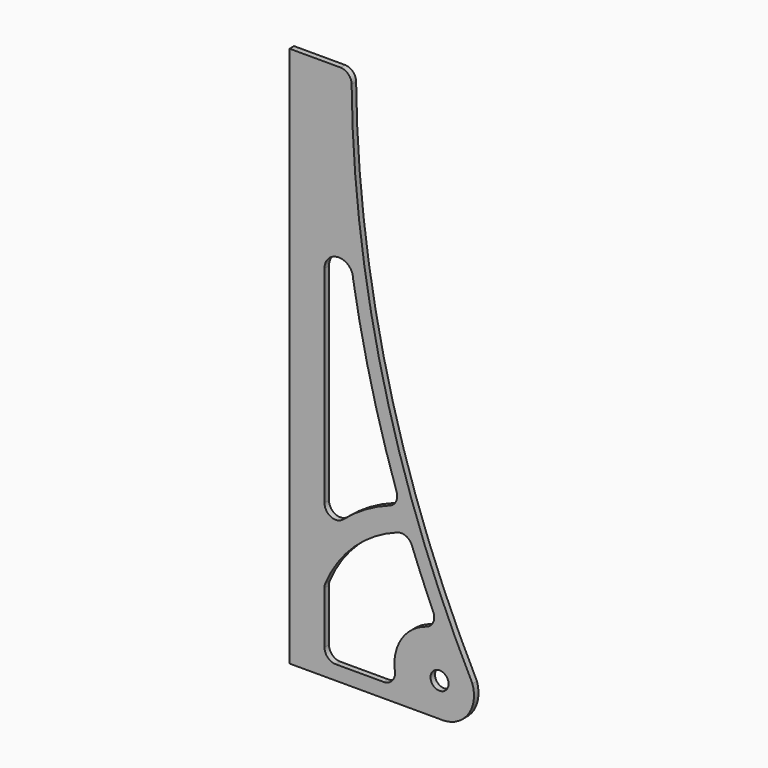
from build123d import *

# Parameters (mm, degrees)
F0_R     = 9.6
F1_DEPTH = 6


# Not quite as in the source:
# - ends of sketch curves that miss each other by under 0.0002 mm in the source are joined


with BuildPart() as f1:
    # F0 (on Front) → F1 (new body)
    with BuildSketch(Plane.XZ):
        with BuildLine():
            Line((-47.37213, 301.952011), (-47.37213, -274.047989))
            Line((-47.37213, -274.047989), (112.22787, -274.047989))
            ThreePointArc((112.22787, -274.047989), (141.6551199022, -261.2050030869), (147.2184839386, -229.5829493499))
            ThreePointArc((147.2184839386, -229.5829493499), (52.6438052156, 22.7491379249), (18.6885296881, 290.0745789968))
            ThreePointArc((18.6885296881, 290.0745789968), (15.1309918192, 298.4805166136), (6.689156, 301.952011))
            Line((6.689156, 301.952011), (-47.37213, 301.952011))
        make_face()
        with BuildLine():
            ThreePointArc((-9.212129772, -186.3147650971), (21.5887703345, -142.086780109), (67.5004011846, -113.8567915125))
            ThreePointArc((67.5004011846, -113.8567915125), (76.5568264391, -114.2337436567), (82.7659804046, -120.8373292291))
            ThreePointArc((82.7659804046, -120.8373292291), (93.8059444216, -148.4795335524), (105.5412180684, -175.8337949696))
            ThreePointArc((105.5412180684, -175.8337949696), (105.4958772539, -185.674964668), (98.1047129391, -192.1727618023))
            ThreePointArc((98.1047129391, -192.1727618023), (71.6615483985, -212.3891980752), (64.7258762989, -244.9444079566))
            ThreePointArc((64.7258762989, -244.9444079566), (61.9247722129, -254.5206063304), (52.850378, -258.668513))
            Line((52.850378, -258.668513), (1.82787, -258.668513))
            ThreePointArc((1.82787, -258.668513), (-6.6574113742, -255.1537943742), (-10.17213, -246.668513))
            Line((-10.17213, -246.668513), (-10.17213, -191.017786))
            ThreePointArc((-10.17213, -191.017786), (-9.9296807015, -188.6177856873), (-9.212129772, -186.3147650971))
        make_face(mode=Mode.SUBTRACT)
        with BuildLine():
            ThreePointArc((19.4670165424, 113.1437789224), (20.0682276951, 110.7367359664), (20.270422, 108.263999))
            ThreePointArc((20.270422, 108.263999), (39.7056889327, 15.1169768951), (66.6000271064, -76.1561949639))
            ThreePointArc((66.6000271064, -76.1561949639), (66.0471154967, -85.2175692958), (59.3066608161, -91.2987274901))
            ThreePointArc((59.3066608161, -91.2987274901), (33.1541685391, -103.5736429809), (9.7135843501, -120.4604844016))
            ThreePointArc((9.7135843501, -120.4604844016), (-3.1406022278, -122.3383987868), (-10.17213, -111.415291))
            Line((-10.17213, -111.415291), (-10.17213, 108.263999))
            ThreePointArc((-10.17213, 108.263999), (2.5764090336, 123.2830806951), (19.4670165424, 113.1437789224))
        make_face(mode=Mode.SUBTRACT)
        with Locations((112.22787, -238.047989)):
            Circle(F0_R, mode=Mode.SUBTRACT)
    extrude(amount=F1_DEPTH)


solid = f1.part
